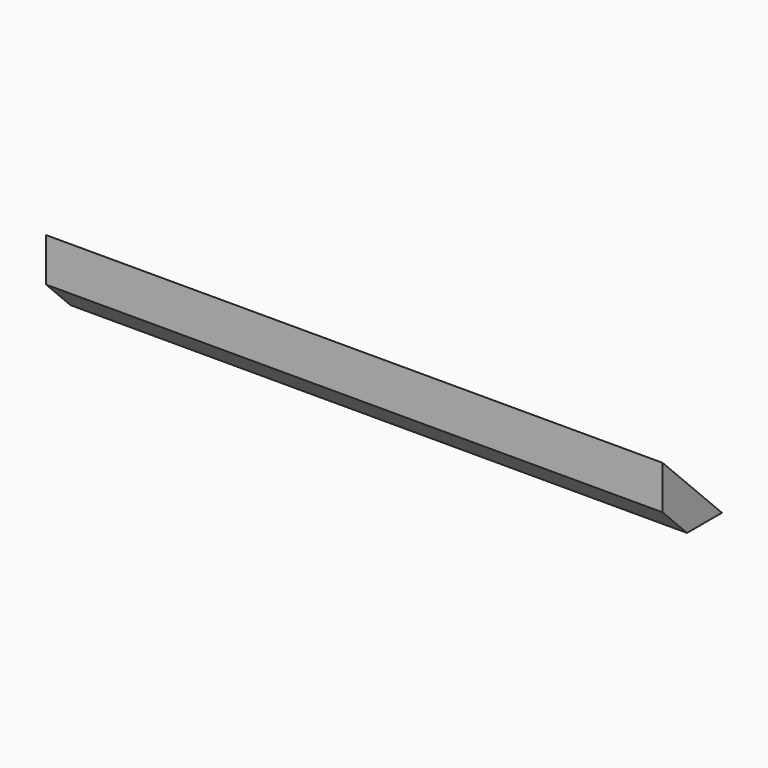
from build123d import *

# Parameters (mm, degrees)
F1_DEPTH = 100
F2_SIZE  = 4.99999


# Not quite as in the source:
# - a fillet or chamfer is up to 0.001 mm smaller than in the source, because OpenCascade refuses the exact size


with BuildPart() as f1:
    # F0 (on Right) → F1 (new body)
    with BuildSketch(Plane.YZ):
        Polygon((7.4991378996, -1.2852627068), (-4.5274403009, 10.7413154936), (-8.0629742068, 7.2057815877), (3.9636039936, -4.8207966127), align=None)
    extrude(amount=F1_DEPTH)

    # F2 (size 5 in the source; OpenCascade refuses exactly that, so slightly less here)
    f2_edges = [f1.edges().sort_by_distance(p)[0] for p in [
        (50, -8.062974, 7.205782),
        (50, 3.963604, -4.820797),
    ]]
    chamfer(f2_edges, length=F2_SIZE)


solid = f1.part
